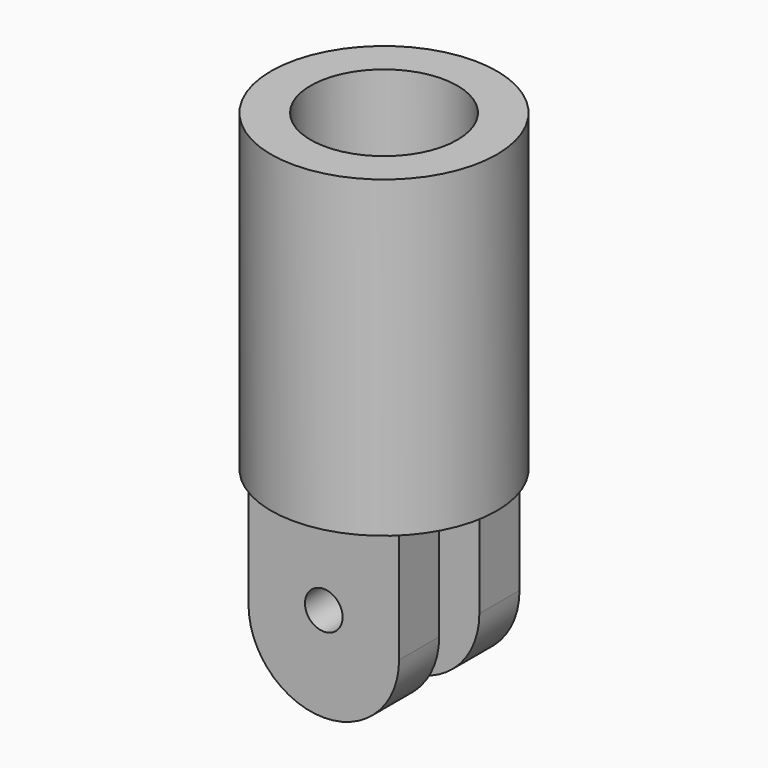
from build123d import *

# Parameters (mm, degrees)
F0_R      = 9
F1_DEPTH  = 25
F2_W      = 12
F2_H      = 4
F3_DEPTH  = 15
F4_R      = 1.5
F5_DEPTH  = 12
F6_R      = 5.99999
F7_R      = 5.85
F8_DEPTH  = 17
F10_DEPTH = 8


# Not quite as in the source:
# - a fillet or chamfer is up to 0.001 mm smaller than in the source, because OpenCascade refuses the exact size


with BuildPart() as f1:
    # F0 (on Top) → F1 (new body)
    with BuildSketch(Plane.XY):
        Circle(F0_R)
    extrude(amount=F1_DEPTH)

    # F2 (on face) → F3 (join)
    with BuildSketch(Plane(origin=(0, 0, 0), x_dir=(1, 0, 0), z_dir=(0, 0, -1))):
        with Locations((0, -4)):
            Rectangle(F2_W, F2_H)
        with Locations((0, 4)):
            Rectangle(F2_W, F2_H)
    extrude(amount=F3_DEPTH)

    # F4 (on face) → F5 (cut, through all)
    with BuildSketch(Plane(origin=(0, 6, 0), x_dir=(-1, 0, 0), z_dir=(0, 1, 0))):
        with Locations((0, -7.464856375)):
            Circle(F4_R)
    extrude(amount=-F5_DEPTH, mode=Mode.SUBTRACT)

    # F6 (radius 6 in the source; OpenCascade refuses exactly that, so slightly less here)
    f6_edges = [f1.edges().sort_by_distance(p)[0] for p in [
        (-6, 4, -15),
        (-6, -4, -15),
        (6, -4, -15),
        (6, 4, -15),
    ]]
    fillet(f6_edges, radius=F6_R)

    # F7 (on face) → F8 (cut)
    with BuildSketch(Plane.XY.offset(25)):
        Circle(F7_R)
    extrude(amount=-F8_DEPTH, mode=Mode.SUBTRACT)

    # F9 (on face) → F10 (cut, through all)
    with BuildSketch(Plane(origin=(0, 0, 0), x_dir=(1, 0, 0), z_dir=(0, 0, -1))):
        with BuildLine():
            ThreePointArc((0, -2), (1.4142135624, -1.4142135624), (2, 0))
            ThreePointArc((2, 0), (1.4142135624, 1.4142135624), (0, 2))
            ThreePointArc((0, 2), (-2, 0), (0, -2))
        make_face()
    extrude(amount=-F10_DEPTH, mode=Mode.SUBTRACT)


solid = f1.part
